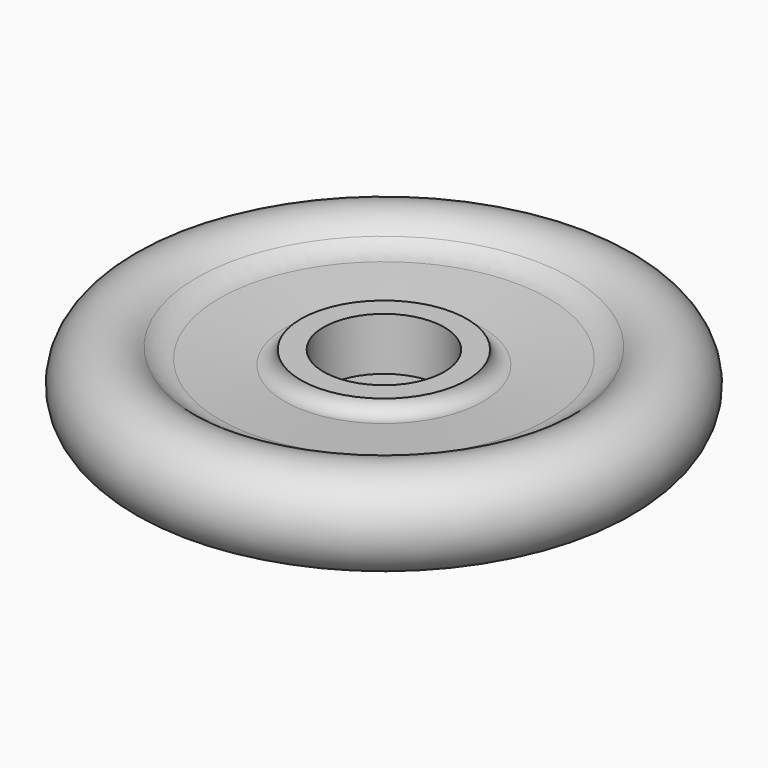
from build123d import *

# Parameters (mm, degrees)
F0_R      = 6
F0_R_2    = 3.5
F5_R      = 5
F7_R      = 4.25
F8_DEPTH  = 10.0181263808
F9_R      = 8
F9_R_2    = 4.25
F10_DEPTH = 7


# Not quite as in the source:
# - a fillet or chamfer that OpenCascade refuses, or shapes differently, is made with other operations: its cross-section is extruded or revolved along the edge and cut away or added


with BuildPart() as f3:
    # F2 (on Front) + F1 (on Front) + F0 (on Front) → F3 (revolve)
    with BuildSketch(Plane.XZ):
        Polygon((0, -3.9828737192), (0, 0), (-11, 0), (-11, -4), align=None)
        Polygon((-11, 0), (0, 0), (0, 4.0171262808), (-11, 4.0171262808), (-11, 4), align=None)
    with BuildSketch(Plane.XZ):
        Polygon((-10.9939463437, 2.0442719534), (-28.9655458182, 3.5265167411), (-28.9655458182, -3.4734832589), (-10.9939463437, -1.9557280466), align=None)
    with BuildSketch(Plane.XZ):
        with Locations((-29, 0)):
            Circle(F0_R)
        with Locations((-29, 0)):
            Circle(F0_R_2, mode=Mode.SUBTRACT)
    revolve(axis=Axis((0, 0, 0.0171262808), (0, 0, -1)))

    # F4: union 

    # F5
    f5_edges = [f3.edges().sort_by_distance(p)[0] for p in [
        (23.866482, 0, 3.105961),
        (23.826857, 0, -3.039506),
    ]]
    fillet(f5_edges, radius=F5_R)

    # F6: fillet of radius 2 on 2 edges, made by hand

    # F6_s1 → F6_t2 (revolve)
    with BuildSketch(Plane.XZ):
        with BuildLine():
            ThreePointArc((-13.1545135111, 2.2224691933), (-11.7100732841, 2.6789883168), (-11, 4.0171262808))
            Line((-11, 4.0171262808), (-10.9601976484, 4.0131547817))
            ThreePointArc((-10.9601976484, 4.0131547817), (-10.96, 3.030948761), (-10.96, 2.0447712412))
            Line((-10.96, 2.0447712412), (-11.0032879186, 2.0049066003))
            Line((-11.0032879186, 2.0049066003), (-13.1578014297, 2.1826045524))
            Line((-13.1578014297, 2.1826045524), (-13.1545135111, 2.2224691933))
        make_face()
    revolve(axis=Axis((0, 0, 2.0447712412), (0, 0, -1)))

    # F6_s3 → F6_t4 (revolve)
    with BuildSketch(Plane.XZ):
        with BuildLine():
            ThreePointArc((-13.1639528708, -2.1389915742), (-11.6915638976, -2.6155299049), (-11, -4))
            Line((-11, -4), (-10.9600870791, -3.9973620561))
            ThreePointArc((-10.9600870791, -3.9973620561), (-10.96, -2.978119648), (-10.96, -1.9562392959))
            Line((-10.96, -1.9562392959), (-11.0033661366, -1.9163811835))
            Line((-11.0033661366, -1.9163811835), (-13.1673190073, -2.0991334618))
            Line((-13.1673190073, -2.0991334618), (-13.1639528708, -2.1389915742))
        make_face()
    revolve(axis=Axis((0, 0, -1.9562392959), (0, 0, -1)))

    # F7 (on face) → F8 (cut, through all)
    with BuildSketch(Plane.XY.offset(4.0171262808)):
        Circle(F7_R)
    extrude(amount=-F8_DEPTH, mode=Mode.SUBTRACT)

    # F9 (on face) → F10 (cut)
    with BuildSketch(Plane.XY.offset(4.0171262808)):
        Circle(F9_R)
        Circle(F9_R_2, mode=Mode.SUBTRACT)
    extrude(amount=-F10_DEPTH, mode=Mode.SUBTRACT)


solid = f3.part
